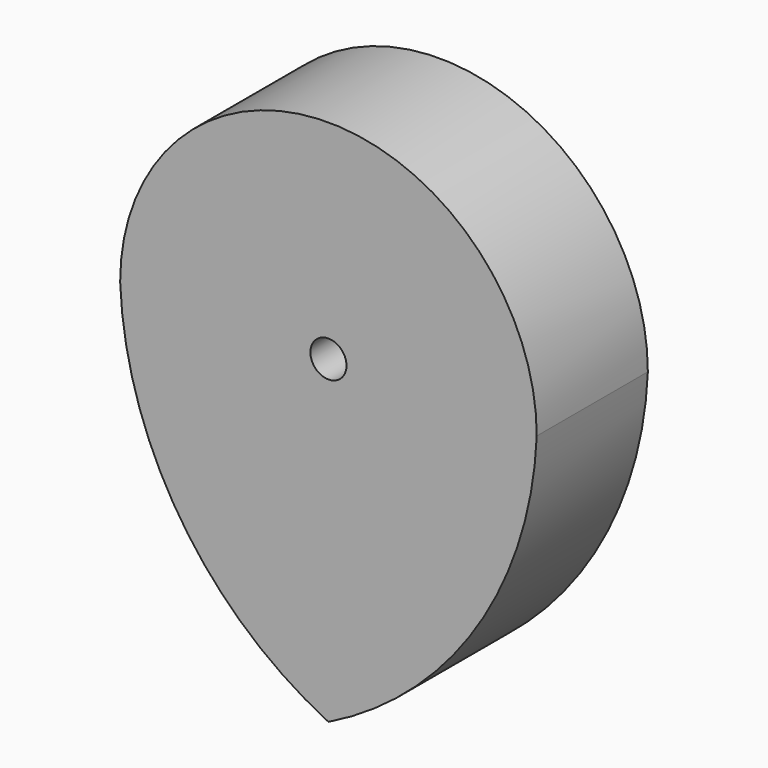
from build123d import *

# Parameters (mm, degrees)
F2_DEPTH = 25.4
F3_R     = 3.302
F4_DEPTH = 25.4


# Not quite as in the source:
# - the program builds the solid bodies; features that only make, move or delete a surface that nothing else refers to are left out


with BuildPart() as f2:
    # F0 (on Front) → F2 (new body)
    with BuildSketch(Plane.XZ):
        with BuildLine():
            ThreePointArc((0, -58.4407677476), (27.0582840041, -34.4413217964), (38.1, 0))
            ThreePointArc((38.1, 0), (0, 38.1), (-38.1, 0))
            ThreePointArc((-38.1, 0), (-27.1159044848, -34.4788870166), (0, -58.4407677476))
        make_face()
    extrude(amount=F2_DEPTH)

    # F3 (on face) → F4 (cut)
    with BuildSketch(Plane(origin=(0, 0, 0), x_dir=(-1, 0, 0), z_dir=(0, 1, 0))):
        Circle(F3_R)
    extrude(amount=-F4_DEPTH, mode=Mode.SUBTRACT)


solid = f2.part
